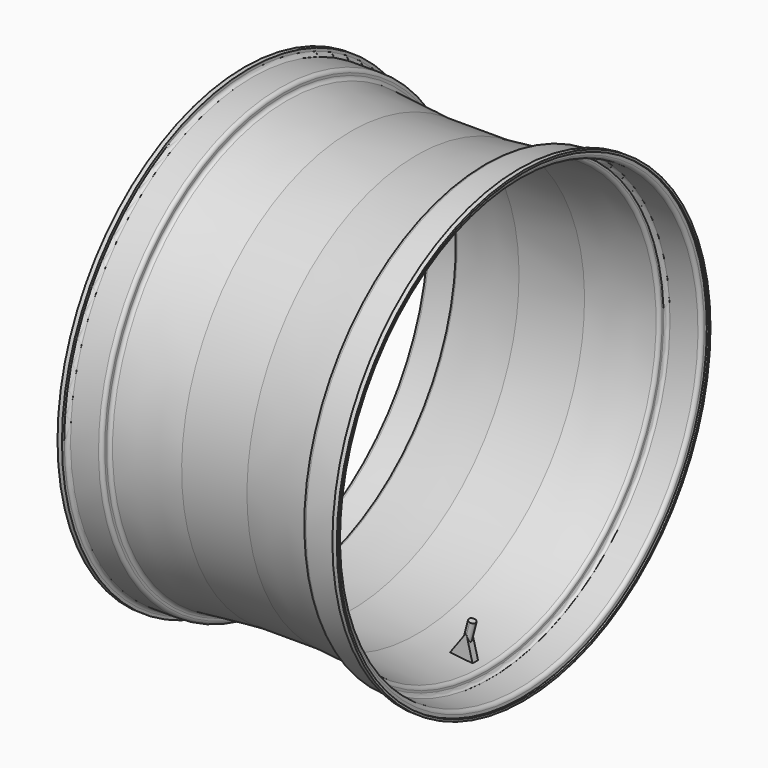
from build123d import *

# Parameters (mm, degrees)
F1_W     = 2.9464
F1_H     = 3.5
F1_H_2   = 2.9464
F6_DEPTH = 5
F7_R     = 4.99999
F8_R     = 5.08
F9_R     = 5.08
F10_R    = 5.08
F11_R    = 5.08
F12_R    = 5.08
F13_R    = 5.08


# Not quite as in the source:
# - a fillet or chamfer is up to 0.001 mm smaller than in the source, because OpenCascade refuses the exact size


with BuildPart() as f3:
    # F0 (on Front) → F3 (revolve)
    with BuildSketch(Plane.XZ):
        Polygon((-123.5, 339.4), (-127, 339.4), (-127, 326.7), (-76.2, 326.7), (-76.2, 314), (25.4, 304.8), (120.6, 304.8), (222.2, 314), (222.2, 326.7), (273, 326.7), (273, 339.4), (269.5, 339.4), (269.5, 330.2), (218.7, 330.2), (218.7, 317.1973907258), (120.4418589413, 308.3), (25.5581410587, 308.3), (-72.7, 317.1973907258), (-72.7, 330.2), (-123.5, 330.2), align=None)
    revolve(axis=Axis((196.6187655926, 0, 0), (1, 0, 0)))

    # F1 (on Front) → F4 (revolve)
    with BuildSketch(Plane.XZ):
        with Locations((-128.4732, 337.65)):
            Rectangle(F1_W, F1_H)
        with Locations((274.4732, 337.9268)):
            Rectangle(F1_W, F1_H_2)
    revolve(axis=Axis((196.6187655926, 0, 0), (1, 0, 0)))

    # F8
    f8_edges = [f3.edges().sort_by_distance(p)[0] for p in [
        (222.2, 0, -314),
        (-76.2, 0, -314),
    ]]
    fillet(f8_edges, radius=F8_R)

    # F9
    f9_edges = [f3.edges().sort_by_distance(p)[0] for p in [
        (222.2, 0, -326.7),
        (-76.2, 0, -326.7),
    ]]
    fillet(f9_edges, radius=F9_R)

    # F10
    f10_edges = [f3.edges().sort_by_distance(p)[0] for p in [
        (-72.7, 0, -330.2),
        (218.7, 0, -330.2),
    ]]
    fillet(f10_edges, radius=F10_R)

    # F11
    f11_edges = [f3.edges().sort_by_distance(p)[0] for p in [
        (273, 0, -326.7),
        (-127, 0, -326.7),
    ]]
    fillet(f11_edges, radius=F11_R)

    # F12
    f12_edges = [f3.edges().sort_by_distance(p)[0] for p in [
        (269.5, 0, -330.2),
        (-123.5, 0, -330.2),
    ]]
    fillet(f12_edges, radius=F12_R)

    # F13
    f13_edges = [f3.edges().sort_by_distance(p)[0] for p in [
        (-72.7, 0, -317.197391),
        (218.7, 0, -317.197391),
    ]]
    fillet(f13_edges, radius=F13_R)


with BuildPart() as f6:
    # F5 (on Front) → F6 (new body, symmetric)
    with BuildSketch(Plane.XZ):
        Polygon((189.974385003, -285.451141925), (171.9667653221, -310.0469287736), (206.225155724, -314.4390183103), (199.5163408505, -288.4944213569), (206.2440047511, -262.4807920826), (196.5625357394, -259.9769634593), align=None)
    extrude(amount=F6_DEPTH, both=True)

    # F7 (radius 5 in the source; OpenCascade refuses exactly that, so slightly less here)
    f7_edges = [f6.edges().sort_by_distance(p)[0] for p in [
        (193.26846, -5, -272.714053),
        (202.880173, -5, -275.487607),
        (202.880173, 5, -275.487607),
        (193.26846, 5, -272.714053),
    ]]
    fillet(f7_edges, radius=F7_R)


solid = Compound([f3.part, f6.part])
